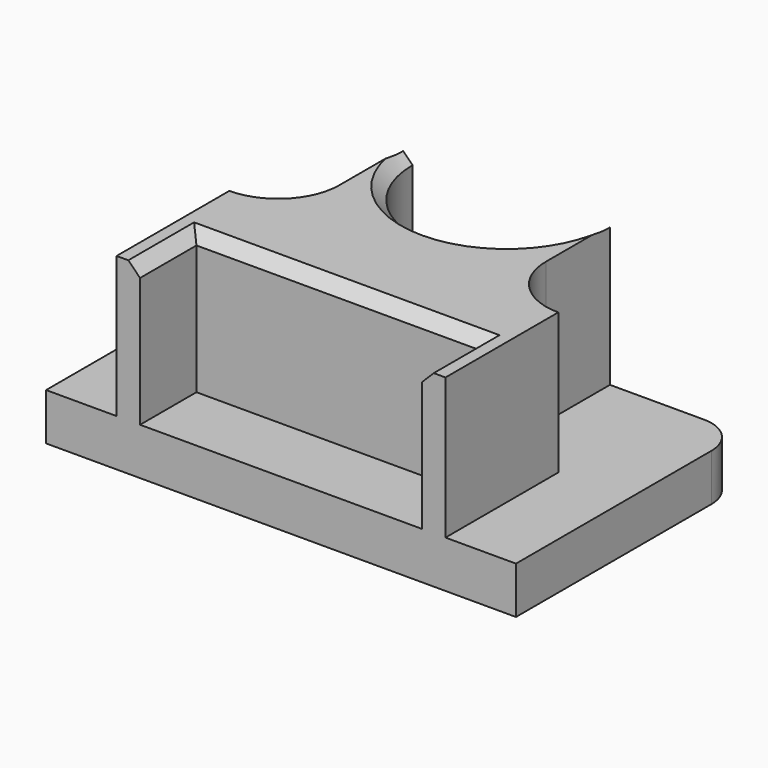
from build123d import *

# Parameters (mm, degrees)
F0_R      = 22.5780805595
F5_DEPTH  = 25.4
F6_W      = 9.525
F6_H      = 38.1
F7_DEPTH  = 19.05
F8_R      = 5.08
F9_W      = 9.525
F9_H      = 38.1
F10_DEPTH = 19.05
F11_W     = 38.1
F11_H     = 9.525
F12_DEPTH = 19.05
F14_R     = 5.08
F13_W     = 8.255
F13_H     = 19.05
F15_DEPTH = 19.05
F16_R     = 8.25499
F17_SIZE  = 1.5875


# Not quite as in the source:
# - a fillet or chamfer is up to 0.001 mm smaller than in the source, because OpenCascade refuses the exact size


with BuildPart() as f2:
    # F2: sweep along a path in F1
    with BuildLine(Plane.XZ) as f2_path:
        Line((0, 0), (57.7025674284, 65.8432990313))
    # F0 (on Top) → F2 (sweep)
    with BuildSketch(Plane.XY):
        with Locations((-2.6368375402, 0)):
            Circle(F0_R)
    sweep(path=f2_path.line)


with BuildPart() as f5:
    # F4 (on Top) → F5 (new body)
    with BuildSketch(Plane.XY):
        with BuildLine():
            Line((-31.75, -19.05), (31.75, -19.05))
            Line((31.75, -19.05), (31.75, 19.05))
            Line((31.75, 19.05), (12.7, 19.05))
            ThreePointArc((12.7, 19.05), (0, 6.35), (-12.7, 19.05))
            Line((-12.7, 19.05), (-31.75, 19.05))
            Line((-31.75, 19.05), (-31.75, -19.05))
        make_face()
    extrude(amount=F5_DEPTH)

    # F6 (on face) → F7 (cut)
    with BuildSketch(Plane.XY.offset(25.4)):
        with Locations((26.9875, 0)):
            Rectangle(F6_W, F6_H)
    extrude(amount=-F7_DEPTH, mode=Mode.SUBTRACT)

    # F8
    f8_edges = [f5.edges().sort_by_distance(p)[0] for p in [
        (31.75, 19.05, 3.175),
    ]]
    fillet(f8_edges, radius=F8_R)

    # F9 (on face) → F10 (cut)
    with BuildSketch(Plane.XY.offset(25.4)):
        with Locations((-26.9875, 0)):
            Rectangle(F9_W, F9_H)
    extrude(amount=-F10_DEPTH, mode=Mode.SUBTRACT)

    # F11 (on face) → F12 (cut)
    with BuildSketch(Plane.XY.offset(25.4)):
        with Locations((0, -14.2875)):
            Rectangle(F11_W, F11_H)
    extrude(amount=-F12_DEPTH, mode=Mode.SUBTRACT)

    # F14
    f14_edges = [f5.edges().sort_by_distance(p)[0] for p in [
        (-31.75, 19.05, 3.175),
    ]]
    fillet(f14_edges, radius=F14_R)

    # F13 (on face) → F15 (cut)
    with BuildSketch(Plane.XY.offset(25.4)):
        with Locations((-18.0975, 9.525)):
            Rectangle(F13_W, F13_H)
        with Locations((18.0975, 9.525)):
            Rectangle(F13_W, F13_H)
    extrude(amount=-F15_DEPTH, mode=Mode.SUBTRACT)

    # F16 (radius 8.255 in the source; OpenCascade refuses exactly that, so slightly less here)
    f16_edges = [f5.edges().sort_by_distance(p)[0] for p in [
        (-13.97, 0, 15.875),
        (13.97, 0, 15.875),
    ]]
    fillet(f16_edges, radius=F16_R)

    # F17
    f17_edges = [f5.edges().sort_by_distance(p)[0] for p in [
        (0, 6.35, 25.4),
        (0, -9.525, 25.4),
        (-19.05, -14.2875, 25.4),
        (19.05, -14.2875, 25.4),
    ]]
    chamfer(f17_edges, length=F17_SIZE)


solid = f5.part
